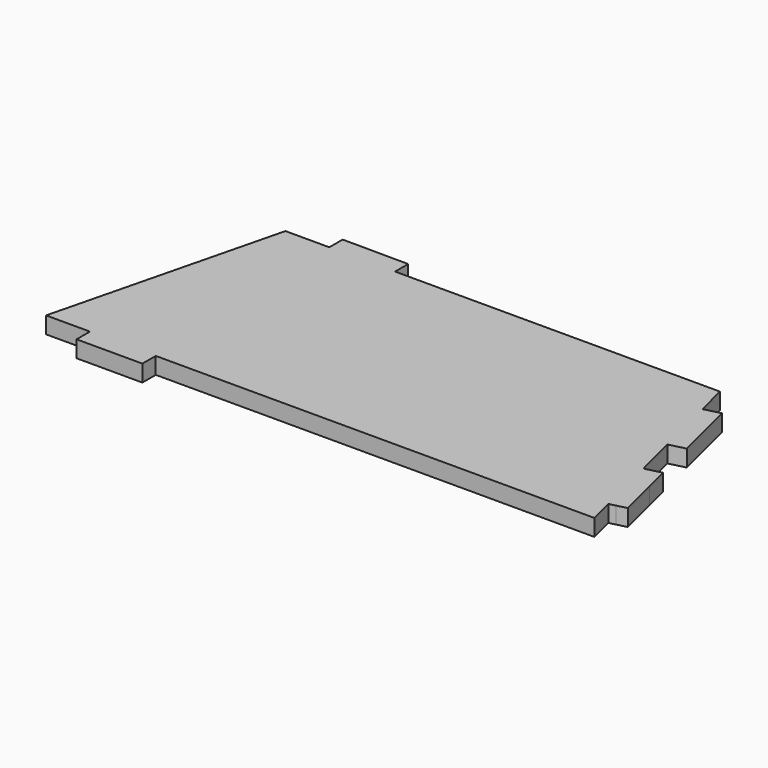
from build123d import *

# Parameters (mm, degrees)
F0_W     = 15
F0_H     = 3.81
F1_DEPTH = 3.81


# Not quite as in the source:
# - a feature names something its author has since deleted; it is built from what else it names


with BuildPart() as f1:
    # F0 (on Top) → F1 (new body)
    with BuildSketch(Plane.XY):
        with Locations((-45, -27.905)):
            Rectangle(F0_W, F0_H)
        Polygon((-37.5, -26), (62.5, -26), (61.059539805, -20.23815922), (57.4215054295, -5.6860217178), (54.9434199682, 4.226320127), (51.3053855927, 18.7784576292), (49.5, 26), (-24.5351687992, 26), (-39.5349438522, 26), (-49.5349438522, 26), (-62.5, -26), (-52.5, -26), align=None)
        Polygon((61.059539805, -20.23815922), (62.5, -19.8780441712), (62.5, -10.2909675664), (61.117748355, -4.7619609864), (57.4215054295, -5.6860217178), align=None)
        Polygon((51.3053855927, 18.7784576292), (54.9434199682, 4.226320127), (58.6396628938, 5.1503808584), (55.0016285183, 19.7025183606), align=None)
        Polygon((62.5, -10.2909675664), (62.5, -19.8780441712), (64.7557827306, -19.3140984886), align=None)
        Polygon((-39.5349438522, 29.81), (-39.5349438522, 26), (-24.5351687992, 26), (-24.5351687992, 29.7278515898), align=None)
    extrude(amount=F1_DEPTH)


solid = f1.part
